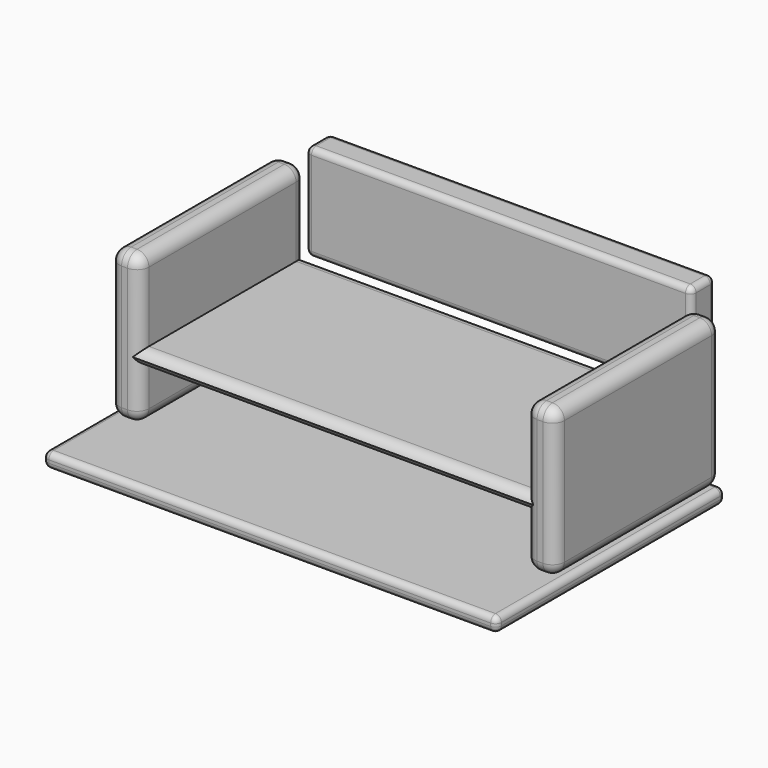
from build123d import *

# Parameters (mm, degrees)
F1_DEPTH      = 88.9
F2_DEPTH      = 6.35
F3_DEPTH      = 6.35
F4_T1_DEPTH   = 17.145
F4_T3_DEPTH   = 165.1
F4_T5_DEPTH   = 2.54
F4_T7_DEPTH   = 53.34
F4_T9_DEPTH   = 29.845
F4_T11_DEPTH  = 2.54
F4_T13_DEPTH  = 78.74
F4_S17_W      = 5.08
F4_S17_H      = 5.08
F4_T18_DEPTH  = 5.08
F4_S23_W      = 5.08
F4_S23_H      = 5.08
F4_T24_DEPTH  = 5.08
F4_S29_W      = 5.08
F4_S29_H      = 5.08
F4_T30_DEPTH  = 5.08
F4_S35_W      = 5.08
F4_S35_H      = 5.08
F4_T36_DEPTH  = 5.08
F4_S41_W      = 5.08
F4_S41_H      = 5.08
F4_T42_DEPTH  = 5.08
F4_S47_W      = 5.08
F4_S47_H      = 5.08
F4_T48_DEPTH  = 5.08
F4_S53_W      = 5.08
F4_S53_H      = 5.08
F4_T54_DEPTH  = 5.08
F4_S59_W      = 5.08
F4_S59_H      = 5.08
F4_T60_DEPTH  = 5.08
F4_S65_W      = 5.08
F4_S65_H      = 5.08
F4_T66_DEPTH  = 5.08
F4_S71_W      = 5.08
F4_S71_H      = 5.08
F4_T72_DEPTH  = 5.08
F4_S77_W      = 5.08
F4_S77_H      = 5.08
F4_T78_DEPTH  = 5.08
F4_S83_W      = 5.08
F4_S83_H      = 5.08
F4_T84_DEPTH  = 5.08
F4_S89_W      = 5.08
F4_S89_H      = 5.08
F4_T90_DEPTH  = 5.08
F4_S95_W      = 5.08
F4_S95_H      = 5.08
F4_T96_DEPTH  = 5.08
F4_S101_W     = 5.08
F4_S101_H     = 5.08
F4_T102_DEPTH = 5.08
F4_S107_W     = 5.08
F4_S107_H     = 5.08
F4_T108_DEPTH = 5.08
F4_T114_DEPTH = 29.845
F4_T119_DEPTH = 29.845
F4_T124_DEPTH = 42.545
F4_T129_DEPTH = 42.545
F4_T134_DEPTH = 29.845
F4_T139_DEPTH = 29.845
F4_T144_DEPTH = 42.545
F4_T149_DEPTH = 42.545
F4_T155_DEPTH = 29.845
F4_T160_DEPTH = 177.8
F4_T167_DEPTH = 177.8
F4_T171_DEPTH = 29.845
F4_T179_DEPTH = 42.545
F4_T184_DEPTH = 177.8
F4_T191_DEPTH = 177.8
F4_T195_DEPTH = 42.545
F4_T203_DEPTH = 29.845
F4_T208_DEPTH = 177.8
F4_T215_DEPTH = 29.845
F4_T220_DEPTH = 177.8
F4_T227_DEPTH = 177.8
F4_T231_DEPTH = 42.545
F4_T239_DEPTH = 42.545
F4_T244_DEPTH = 177.8
F5_DEPTH      = 122.15182
F6_DEPTH      = 8.30271
F7_DEPTH      = 8.03557
F8_R          = 2.54
F9_DEPTH      = 12.7
F10_R         = 2.54


# Not quite as in the source:
# - a fillet or chamfer that OpenCascade refuses, or shapes differently, is made with other operations: its cross-section is extruded or revolved along the edge and cut away or added


with BuildPart() as f1:
    # F0 (on Front) → F1 (new body)
    with BuildSketch(Plane.XZ):
        Polygon((82.55, -28.575), (88.9, -28.575), (88.9, 34.925), (82.55, 34.925), (82.55, 0), (-82.55, 0), (-82.55, 34.925), (-88.9, 34.925), (-88.9, -28.575), (-82.55, -28.575), (-82.55, -6.35), (82.55, -6.35), align=None)
    extrude(amount=F1_DEPTH)

    # F2 (add): a face of the model
    f2_faces = [f1.faces().sort_by_distance(p)[0] for p in [
        (-88.9, -44.45, 3.175),
    ]]
    extrude(f2_faces, amount=F2_DEPTH)

    # F3 (add): a face of the model
    f3_faces = [f1.faces().sort_by_distance(p)[0] for p in [
        (88.9, -44.45, 3.175),
    ]]
    extrude(f3_faces, amount=F3_DEPTH)

    # F4: fillet of radius 5.08 on 32 edges, made by hand

    # F4_s2 → F4_t1 (cut)
    with BuildSketch(Plane.XY.offset(-23.495)):
        with BuildLine():
            ThreePointArc((-82.55, -83.82), (-84.0378975516, -87.4121024484), (-87.63, -88.9))
            Line((-87.63, -88.9), (-82.55, -88.9))
            Line((-82.55, -88.9), (-82.55, -83.82))
        make_face()
        with BuildLine():
            ThreePointArc((87.63, -88.9), (84.0378975516, -87.4121024484), (82.55, -83.82))
            Line((82.55, -83.82), (82.55, -88.9))
            Line((82.55, -88.9), (87.63, -88.9))
        make_face()
        with BuildLine():
            ThreePointArc((-82.55, -5.08), (-84.0378975516, -1.4878975516), (-87.63, 0))
            Line((-87.63, 0), (-82.55, 0))
            Line((-82.55, 0), (-82.55, -5.08))
        make_face()
        with BuildLine():
            ThreePointArc((82.55, -5.08), (84.0378975516, -1.4878975516), (87.63, 0))
            Line((87.63, 0), (82.55, 0))
            Line((82.55, 0), (82.55, -5.08))
        make_face()
    extrude(amount=F4_T1_DEPTH, mode=Mode.SUBTRACT)

    # F4_s4 → F4_t3 (cut)
    with BuildSketch(Plane.YZ.offset(-82.55)):
        with BuildLine():
            ThreePointArc((-88.9, -1.27), (-87.4121024484, -4.8621024484), (-83.82, -6.35))
            Line((-83.82, -6.35), (-88.9, -6.35))
            Line((-88.9, -6.35), (-88.9, -1.27))
        make_face()
        with BuildLine():
            ThreePointArc((-88.9, -5.08), (-87.4121024484, -1.4878975516), (-83.82, 0))
            Line((-83.82, 0), (-88.9, 0))
            Line((-88.9, 0), (-88.9, -5.08))
        make_face()
        with BuildLine():
            ThreePointArc((0, -1.27), (-1.4878975516, -4.8621024484), (-5.08, -6.35))
            Line((-5.08, -6.35), (0, -6.35))
            Line((0, -6.35), (0, -1.27))
        make_face()
        with BuildLine():
            ThreePointArc((-5.08, 0), (-1.4878975516, -1.4878975516), (0, -5.08))
            Line((0, -5.08), (0, 0))
            Line((0, 0), (-5.08, 0))
        make_face()
    extrude(amount=F4_T3_DEPTH, mode=Mode.SUBTRACT)

    # F4_s6 → F4_t5 (cut)
    with BuildSketch(Plane.YZ.offset(87.63)):
        with BuildLine():
            ThreePointArc((-88.9, -23.495), (-87.4121024484, -27.0871024484), (-83.82, -28.575))
            Line((-83.82, -28.575), (-88.9, -28.575))
            Line((-88.9, -28.575), (-88.9, -23.495))
        make_face()
        with BuildLine():
            ThreePointArc((-88.9, 29.845), (-87.4121024484, 33.4371024484), (-83.82, 34.925))
            Line((-83.82, 34.925), (-88.9, 34.925))
            Line((-88.9, 34.925), (-88.9, 29.845))
        make_face()
        with BuildLine():
            ThreePointArc((-5.08, 34.925), (-1.4878975516, 33.4371024484), (0, 29.845))
            Line((0, 29.845), (0, 34.925))
            Line((0, 34.925), (-5.08, 34.925))
        make_face()
        with BuildLine():
            ThreePointArc((-5.08, -28.575), (-1.4878975516, -27.0871024484), (0, -23.495))
            Line((0, -23.495), (0, -28.575))
            Line((0, -28.575), (-5.08, -28.575))
        make_face()
    extrude(amount=F4_T5_DEPTH, mode=Mode.SUBTRACT)

    # F4_s8 → F4_t7 (cut)
    with BuildSketch(Plane.XY.offset(-23.495)):
        with BuildLine():
            ThreePointArc((90.17, -88.9), (93.7621024484, -87.4121024484), (95.25, -83.82))
            Line((95.25, -83.82), (95.25, -88.9))
            Line((95.25, -88.9), (90.17, -88.9))
        make_face()
        with BuildLine():
            ThreePointArc((-90.17, -88.9), (-93.7621024484, -87.4121024484), (-95.25, -83.82))
            Line((-95.25, -83.82), (-95.25, -88.9))
            Line((-95.25, -88.9), (-90.17, -88.9))
        make_face()
        with BuildLine():
            ThreePointArc((95.25, -5.08), (93.7621024484, -1.4878975516), (90.17, 0))
            Line((90.17, 0), (95.25, 0))
            Line((95.25, 0), (95.25, -5.08))
        make_face()
        with BuildLine():
            ThreePointArc((-95.25, -5.08), (-93.7621024484, -1.4878975516), (-90.17, 0))
            Line((-90.17, 0), (-95.25, 0))
            Line((-95.25, 0), (-95.25, -5.08))
        make_face()
    extrude(amount=F4_T7_DEPTH, mode=Mode.SUBTRACT)

    # F4_s10 → F4_t9 (cut)
    with BuildSketch(Plane.XY):
        with BuildLine():
            ThreePointArc((87.63, -88.9), (84.0378975516, -87.4121024484), (82.55, -83.82))
            Line((82.55, -83.82), (82.55, -88.9))
            Line((82.55, -88.9), (87.63, -88.9))
        make_face()
        with BuildLine():
            ThreePointArc((-87.63, -88.9), (-84.0378975516, -87.4121024484), (-82.55, -83.82))
            Line((-82.55, -83.82), (-82.55, -88.9))
            Line((-82.55, -88.9), (-87.63, -88.9))
        make_face()
        with BuildLine():
            ThreePointArc((82.55, -5.08), (84.0378975516, -1.4878975516), (87.63, 0))
            Line((87.63, 0), (82.55, 0))
            Line((82.55, 0), (82.55, -5.08))
        make_face()
        with BuildLine():
            ThreePointArc((-82.55, -5.08), (-84.0378975516, -1.4878975516), (-87.63, 0))
            Line((-87.63, 0), (-82.55, 0))
            Line((-82.55, 0), (-82.55, -5.08))
        make_face()
    extrude(amount=F4_T9_DEPTH, mode=Mode.SUBTRACT)

    # F4_s12 → F4_t11 (cut)
    with BuildSketch(Plane.YZ.offset(-90.17)):
        with BuildLine():
            ThreePointArc((-88.9, 29.845), (-87.4121024484, 33.4371024484), (-83.82, 34.925))
            Line((-83.82, 34.925), (-88.9, 34.925))
            Line((-88.9, 34.925), (-88.9, 29.845))
        make_face()
        with BuildLine():
            ThreePointArc((-88.9, -23.495), (-87.4121024484, -27.0871024484), (-83.82, -28.575))
            Line((-83.82, -28.575), (-88.9, -28.575))
            Line((-88.9, -28.575), (-88.9, -23.495))
        make_face()
        with BuildLine():
            ThreePointArc((-5.08, 34.925), (-1.4878975516, 33.4371024484), (0, 29.845))
            Line((0, 29.845), (0, 34.925))
            Line((0, 34.925), (-5.08, 34.925))
        make_face()
        with BuildLine():
            ThreePointArc((0, -23.495), (-1.4878975516, -27.0871024484), (-5.08, -28.575))
            Line((-5.08, -28.575), (0, -28.575))
            Line((0, -28.575), (0, -23.495))
        make_face()
    extrude(amount=F4_T11_DEPTH, mode=Mode.SUBTRACT)

    # F4_s14 → F4_t13 (cut)
    with BuildSketch(Plane.XZ.offset(5.08)):
        with BuildLine():
            ThreePointArc((-87.63, 34.925), (-84.0378975516, 33.4371024484), (-82.55, 29.845))
            Line((-82.55, 29.845), (-82.55, 34.925))
            Line((-82.55, 34.925), (-87.63, 34.925))
        make_face()
        with BuildLine():
            ThreePointArc((-95.25, 29.845), (-93.7621024484, 33.4371024484), (-90.17, 34.925))
            Line((-90.17, 34.925), (-95.25, 34.925))
            Line((-95.25, 34.925), (-95.25, 29.845))
        make_face()
        with BuildLine():
            ThreePointArc((82.55, 29.845), (84.0378975516, 33.4371024484), (87.63, 34.925))
            Line((87.63, 34.925), (82.55, 34.925))
            Line((82.55, 34.925), (82.55, 29.845))
        make_face()
        with BuildLine():
            ThreePointArc((90.17, 34.925), (93.7621024484, 33.4371024484), (95.25, 29.845))
            Line((95.25, 29.845), (95.25, 34.925))
            Line((95.25, 34.925), (90.17, 34.925))
        make_face()
        with BuildLine():
            ThreePointArc((87.63, -28.575), (84.0378975516, -27.0871024484), (82.55, -23.495))
            Line((82.55, -23.495), (82.55, -28.575))
            Line((82.55, -28.575), (87.63, -28.575))
        make_face()
        with BuildLine():
            ThreePointArc((95.25, -23.495), (93.7621024484, -27.0871024484), (90.17, -28.575))
            Line((90.17, -28.575), (95.25, -28.575))
            Line((95.25, -28.575), (95.25, -23.495))
        make_face()
        with BuildLine():
            ThreePointArc((-82.55, -23.495), (-84.0378975516, -27.0871024484), (-87.63, -28.575))
            Line((-87.63, -28.575), (-82.55, -28.575))
            Line((-82.55, -28.575), (-82.55, -23.495))
        make_face()
        with BuildLine():
            ThreePointArc((-95.25, -23.495), (-93.7621024484, -27.0871024484), (-90.17, -28.575))
            Line((-90.17, -28.575), (-95.25, -28.575))
            Line((-95.25, -28.575), (-95.25, -23.495))
        make_face()
    extrude(amount=F4_T13_DEPTH, mode=Mode.SUBTRACT)


with BuildPart() as f4_tool16:
    # F4_s17 → F4_t18 (new body)
    with BuildSketch(Plane.YZ.offset(-87.63)):
        with Locations((-86.36, -26.035)):
            Rectangle(F4_S17_W, F4_S17_H)
    extrude(amount=F4_T18_DEPTH)

    # F4_s19 → F4_t20 (revolve, cut)
    with BuildSketch(Plane(origin=(-87.63, -83.82, -23.495), x_dir=(0, 0.7071067812, 0.7071067812), z_dir=(0, 0.7071067812, -0.7071067812))):
        with BuildLine():
            ThreePointArc((0, -5.08), (5.08, 0), (0, 5.08))
            Line((0, 5.08), (0, -5.08))
        make_face()
    revolve(axis=Axis((-87.63, -83.82, -23.495), (1, 0, 0)), mode=Mode.SUBTRACT)


with BuildPart() as f1_1:
    add(f1.part)

    # F4_t15: cut F4_tool16
    add(f4_tool16.part, mode=Mode.SUBTRACT)


with BuildPart() as f4_tool22:
    # F4_s23 → F4_t24 (new body)
    with BuildSketch(Plane.XZ.offset(83.82)):
        with Locations((85.09, -26.035)):
            Rectangle(F4_S23_W, F4_S23_H)
    extrude(amount=F4_T24_DEPTH)

    # F4_s25 → F4_t26 (revolve, cut)
    with BuildSketch(Plane(origin=(87.63, -83.82, -23.495), x_dir=(0.7071067812, 0, 0.7071067812), z_dir=(0.7071067812, 0, -0.7071067812))):
        with BuildLine():
            ThreePointArc((0, -5.08), (5.08, 0), (0, 5.08))
            Line((0, 5.08), (0, -5.08))
        make_face()
    revolve(axis=Axis((87.63, -83.82, -23.495), (0, -1, 0)), mode=Mode.SUBTRACT)


with BuildPart() as f1_2:
    add(f1_1.part)

    # F4_t21: cut F4_tool22
    add(f4_tool22.part, mode=Mode.SUBTRACT)


with BuildPart() as f4_tool28:
    # F4_s29 → F4_t30 (new body)
    with BuildSketch(Plane.YZ.offset(90.17)):
        with Locations((-86.36, -26.035)):
            Rectangle(F4_S29_W, F4_S29_H)
    extrude(amount=F4_T30_DEPTH)

    # F4_s31 → F4_t32 (revolve, cut)
    with BuildSketch(Plane(origin=(90.17, -83.82, -23.495), x_dir=(0, 0.7071067812, 0.7071067812), z_dir=(0, 0.7071067812, -0.7071067812))):
        with BuildLine():
            ThreePointArc((0, -5.08), (5.08, 0), (0, 5.08))
            Line((0, 5.08), (0, -5.08))
        make_face()
    revolve(axis=Axis((90.17, -83.82, -23.495), (1, 0, 0)), mode=Mode.SUBTRACT)


with BuildPart() as f1_3:
    add(f1_2.part)

    # F4_t27: cut F4_tool28
    add(f4_tool28.part, mode=Mode.SUBTRACT)


with BuildPart() as f4_tool34:
    # F4_s35 → F4_t36 (new body)
    with BuildSketch(Plane.YZ.offset(90.17)):
        with Locations((-86.36, 32.385)):
            Rectangle(F4_S35_W, F4_S35_H)
    extrude(amount=F4_T36_DEPTH)

    # F4_s37 → F4_t38 (revolve, cut)
    with BuildSketch(Plane(origin=(90.17, -83.82, 29.845), x_dir=(0, 0.7071067812, -0.7071067812), z_dir=(0, -0.7071067812, -0.7071067812))):
        with BuildLine():
            ThreePointArc((0, -5.08), (5.08, 0), (0, 5.08))
            Line((0, 5.08), (0, -5.08))
        make_face()
    revolve(axis=Axis((90.17, -83.82, 29.845), (1, 0, 0)), mode=Mode.SUBTRACT)


with BuildPart() as f1_4:
    add(f1_3.part)

    # F4_t33: cut F4_tool34
    add(f4_tool34.part, mode=Mode.SUBTRACT)


with BuildPart() as f4_tool40:
    # F4_s41 → F4_t42 (new body)
    with BuildSketch(Plane.XZ.offset(83.82)):
        with Locations((85.09, 32.385)):
            Rectangle(F4_S41_W, F4_S41_H)
    extrude(amount=F4_T42_DEPTH)

    # F4_s43 → F4_t44 (revolve, cut)
    with BuildSketch(Plane(origin=(87.63, -83.82, 29.845), x_dir=(0.7071067812, 0, -0.7071067812), z_dir=(-0.7071067812, 0, -0.7071067812))):
        with BuildLine():
            ThreePointArc((0, -5.08), (5.08, 0), (0, 5.08))
            Line((0, 5.08), (0, -5.08))
        make_face()
    revolve(axis=Axis((87.63, -83.82, 29.845), (0, -1, 0)), mode=Mode.SUBTRACT)


with BuildPart() as f1_5:
    add(f1_4.part)

    # F4_t39: cut F4_tool40
    add(f4_tool40.part, mode=Mode.SUBTRACT)


with BuildPart() as f4_tool46:
    # F4_s47 → F4_t48 (new body)
    with BuildSketch(Plane.XZ.offset(83.82)):
        with Locations((-85.09, 32.385)):
            Rectangle(F4_S47_W, F4_S47_H)
    extrude(amount=F4_T48_DEPTH)

    # F4_s49 → F4_t50 (revolve, cut)
    with BuildSketch(Plane(origin=(-87.63, -83.82, 29.845), x_dir=(-0.7071067812, 0, -0.7071067812), z_dir=(-0.7071067812, 0, 0.7071067812))):
        with BuildLine():
            ThreePointArc((0, -5.08), (5.08, 0), (0, 5.08))
            Line((0, 5.08), (0, -5.08))
        make_face()
    revolve(axis=Axis((-87.63, -83.82, 29.845), (0, -1, 0)), mode=Mode.SUBTRACT)


with BuildPart() as f1_6:
    add(f1_5.part)

    # F4_t45: cut F4_tool46
    add(f4_tool46.part, mode=Mode.SUBTRACT)


with BuildPart() as f4_tool52:
    # F4_s53 → F4_t54 (new body)
    with BuildSketch(Plane.XZ.offset(83.82)):
        with Locations((-92.71, 32.385)):
            Rectangle(F4_S53_W, F4_S53_H)
    extrude(amount=F4_T54_DEPTH)

    # F4_s55 → F4_t56 (revolve, cut)
    with BuildSketch(Plane(origin=(-90.17, -83.82, 29.845), x_dir=(0.7071067812, 0, -0.7071067812), z_dir=(-0.7071067812, 0, -0.7071067812))):
        with BuildLine():
            ThreePointArc((0, -5.08), (5.08, 0), (0, 5.08))
            Line((0, 5.08), (0, -5.08))
        make_face()
    revolve(axis=Axis((-90.17, -83.82, 29.845), (0, -1, 0)), mode=Mode.SUBTRACT)


with BuildPart() as f1_7:
    add(f1_6.part)

    # F4_t51: cut F4_tool52
    add(f4_tool52.part, mode=Mode.SUBTRACT)


with BuildPart() as f4_tool58:
    # F4_s59 → F4_t60 (new body)
    with BuildSketch(Plane.XZ.offset(83.82)):
        with Locations((-92.71, -26.035)):
            Rectangle(F4_S59_W, F4_S59_H)
    extrude(amount=F4_T60_DEPTH)

    # F4_s61 → F4_t62 (revolve, cut)
    with BuildSketch(Plane(origin=(-90.17, -83.82, -23.495), x_dir=(0.7071067812, 0, 0.7071067812), z_dir=(0.7071067812, 0, -0.7071067812))):
        with BuildLine():
            ThreePointArc((0, -5.08), (5.08, 0), (0, 5.08))
            Line((0, 5.08), (0, -5.08))
        make_face()
    revolve(axis=Axis((-90.17, -83.82, -23.495), (0, -1, 0)), mode=Mode.SUBTRACT)


with BuildPart() as f1_8:
    add(f1_7.part)

    # F4_t57: cut F4_tool58
    add(f4_tool58.part, mode=Mode.SUBTRACT)


with BuildPart() as f4_tool64:
    # F4_s65 → F4_t66 (new body)
    with BuildSketch(Plane.XZ.offset(5.08)):
        with Locations((-85.09, 32.385)):
            Rectangle(F4_S65_W, F4_S65_H)
    extrude(amount=-F4_T66_DEPTH)

    # F4_s67 → F4_t68 (revolve, cut)
    with BuildSketch(Plane(origin=(-87.63, -5.08, 29.845), x_dir=(-0.7071067812, 0, -0.7071067812), z_dir=(0.7071067812, 0, -0.7071067812))):
        with BuildLine():
            ThreePointArc((0, -5.08), (5.08, 0), (0, 5.08))
            Line((0, 5.08), (0, -5.08))
        make_face()
    revolve(axis=Axis((-87.63, -5.08, 29.845), (0, 1, 0)), mode=Mode.SUBTRACT)


with BuildPart() as f1_9:
    add(f1_8.part)

    # F4_t63: cut F4_tool64
    add(f4_tool64.part, mode=Mode.SUBTRACT)


with BuildPart() as f4_tool70:
    # F4_s71 → F4_t72 (new body)
    with BuildSketch(Plane.XZ.offset(5.08)):
        with Locations((-92.71, 32.385)):
            Rectangle(F4_S71_W, F4_S71_H)
    extrude(amount=-F4_T72_DEPTH)

    # F4_s73 → F4_t74 (revolve, cut)
    with BuildSketch(Plane(origin=(-90.17, -5.08, 29.845), x_dir=(0.7071067812, 0, -0.7071067812), z_dir=(0.7071067812, 0, 0.7071067812))):
        with BuildLine():
            ThreePointArc((0, -5.08), (5.08, 0), (0, 5.08))
            Line((0, 5.08), (0, -5.08))
        make_face()
    revolve(axis=Axis((-90.17, -5.08, 29.845), (0, 1, 0)), mode=Mode.SUBTRACT)


with BuildPart() as f1_10:
    add(f1_9.part)

    # F4_t69: cut F4_tool70
    add(f4_tool70.part, mode=Mode.SUBTRACT)


with BuildPart() as f4_tool76:
    # F4_s77 → F4_t78 (new body)
    with BuildSketch(Plane.XZ.offset(5.08)):
        with Locations((85.09, 32.385)):
            Rectangle(F4_S77_W, F4_S77_H)
    extrude(amount=-F4_T78_DEPTH)

    # F4_s79 → F4_t80 (revolve, cut)
    with BuildSketch(Plane(origin=(87.63, -5.08, 29.845), x_dir=(0.7071067812, 0, -0.7071067812), z_dir=(0.7071067812, 0, 0.7071067812))):
        with BuildLine():
            ThreePointArc((0, -5.08), (5.08, 0), (0, 5.08))
            Line((0, 5.08), (0, -5.08))
        make_face()
    revolve(axis=Axis((87.63, -5.08, 29.845), (0, 1, 0)), mode=Mode.SUBTRACT)


with BuildPart() as f1_11:
    add(f1_10.part)

    # F4_t75: cut F4_tool76
    add(f4_tool76.part, mode=Mode.SUBTRACT)


with BuildPart() as f4_tool82:
    # F4_s83 → F4_t84 (new body)
    with BuildSketch(Plane.YZ.offset(90.17)):
        with Locations((-2.54, 32.385)):
            Rectangle(F4_S83_W, F4_S83_H)
    extrude(amount=F4_T84_DEPTH)

    # F4_s85 → F4_t86 (revolve, cut)
    with BuildSketch(Plane(origin=(90.17, -5.08, 29.845), x_dir=(0, -0.7071067812, -0.7071067812), z_dir=(0, -0.7071067812, 0.7071067812))):
        with BuildLine():
            ThreePointArc((0, -5.08), (5.08, 0), (0, 5.08))
            Line((0, 5.08), (0, -5.08))
        make_face()
    revolve(axis=Axis((90.17, -5.08, 29.845), (1, 0, 0)), mode=Mode.SUBTRACT)


with BuildPart() as f1_12:
    add(f1_11.part)

    # F4_t81: cut F4_tool82
    add(f4_tool82.part, mode=Mode.SUBTRACT)


with BuildPart() as f4_tool88:
    # F4_s89 → F4_t90 (new body)
    with BuildSketch(Plane.XY.offset(-23.495)):
        with Locations((85.09, -2.54)):
            Rectangle(F4_S89_W, F4_S89_H)
    extrude(amount=-F4_T90_DEPTH)

    # F4_s91 → F4_t92 (revolve, cut)
    with BuildSketch(Plane(origin=(87.63, -5.08, -23.495), x_dir=(0.7071067812, -0.7071067812, 0), z_dir=(0.7071067812, 0.7071067812, 0))):
        with BuildLine():
            ThreePointArc((0, -5.08), (5.08, 0), (0, 5.08))
            Line((0, 5.08), (0, -5.08))
        make_face()
    revolve(axis=Axis((87.63, -5.08, -23.495), (0, 0, -1)), mode=Mode.SUBTRACT)


with BuildPart() as f1_13:
    add(f1_12.part)

    # F4_t87: cut F4_tool88
    add(f4_tool88.part, mode=Mode.SUBTRACT)


with BuildPart() as f4_tool94:
    # F4_s95 → F4_t96 (new body)
    with BuildSketch(Plane.YZ.offset(90.17)):
        with Locations((-2.54, -26.035)):
            Rectangle(F4_S95_W, F4_S95_H)
    extrude(amount=F4_T96_DEPTH)

    # F4_s97 → F4_t98 (revolve, cut)
    with BuildSketch(Plane(origin=(90.17, -5.08, -23.495), x_dir=(0, -0.7071067812, 0.7071067812), z_dir=(0, 0.7071067812, 0.7071067812))):
        with BuildLine():
            ThreePointArc((0, -5.08), (5.08, 0), (0, 5.08))
            Line((0, 5.08), (0, -5.08))
        make_face()
    revolve(axis=Axis((90.17, -5.08, -23.495), (1, 0, 0)), mode=Mode.SUBTRACT)


with BuildPart() as f1_14:
    add(f1_13.part)

    # F4_t93: cut F4_tool94
    add(f4_tool94.part, mode=Mode.SUBTRACT)


with BuildPart() as f4_tool100:
    # F4_s101 → F4_t102 (new body)
    with BuildSketch(Plane.YZ.offset(-87.63)):
        with Locations((-2.54, -26.035)):
            Rectangle(F4_S101_W, F4_S101_H)
    extrude(amount=F4_T102_DEPTH)

    # F4_s103 → F4_t104 (revolve, cut)
    with BuildSketch(Plane(origin=(-87.63, -5.08, -23.495), x_dir=(0, -0.7071067812, 0.7071067812), z_dir=(0, 0.7071067812, 0.7071067812))):
        with BuildLine():
            ThreePointArc((0, -5.08), (5.08, 0), (0, 5.08))
            Line((0, 5.08), (0, -5.08))
        make_face()
    revolve(axis=Axis((-87.63, -5.08, -23.495), (1, 0, 0)), mode=Mode.SUBTRACT)


with BuildPart() as f1_15:
    add(f1_14.part)

    # F4_t99: cut F4_tool100
    add(f4_tool100.part, mode=Mode.SUBTRACT)


with BuildPart() as f4_tool106:
    # F4_s107 → F4_t108 (new body)
    with BuildSketch(Plane.YZ.offset(-90.17)):
        with Locations((-2.54, -26.035)):
            Rectangle(F4_S107_W, F4_S107_H)
    extrude(amount=-F4_T108_DEPTH)

    # F4_s109 → F4_t110 (revolve, cut)
    with BuildSketch(Plane(origin=(-90.17, -5.08, -23.495), x_dir=(0, -0.7071067812, 0.7071067812), z_dir=(0, -0.7071067812, -0.7071067812))):
        with BuildLine():
            ThreePointArc((0, -5.08), (5.08, 0), (0, 5.08))
            Line((0, 5.08), (0, -5.08))
        make_face()
    revolve(axis=Axis((-90.17, -5.08, -23.495), (-1, 0, 0)), mode=Mode.SUBTRACT)


with BuildPart() as f1_16:
    add(f1_15.part)

    # F4_t105: cut F4_tool106
    add(f4_tool106.part, mode=Mode.SUBTRACT)


with BuildPart() as f4_tool112:
    # F4_s113 → F4_t114 (new body)
    with BuildSketch(Plane.XY.offset(-23.495)):
        with BuildLine():
            ThreePointArc((-82.55, -83.82), (-84.0378975516, -87.4121024484), (-87.63, -88.9))
            Line((-87.63, -88.9), (-82.55, -88.9))
            Line((-82.55, -88.9), (-82.55, -83.82))
        make_face()
    extrude(amount=F4_T114_DEPTH)

    split(bisect_by=Plane.XY, keep=Keep.TOP)


with BuildPart() as f1_17:
    add(f1_16.part)

    # F4_t111: cut F4_tool112
    add(f4_tool112.part, mode=Mode.SUBTRACT)


with BuildPart() as f4_tool117:
    # F4_s118 → F4_t119 (new body)
    with BuildSketch(Plane.XY.offset(6.35)):
        with BuildLine():
            ThreePointArc((87.63, -88.9), (84.0378975516, -87.4121024484), (82.55, -83.82))
            Line((82.55, -83.82), (82.55, -88.9))
            Line((82.55, -88.9), (87.63, -88.9))
        make_face()
    extrude(amount=-F4_T119_DEPTH)

    split(bisect_by=Plane.XY, keep=Keep.TOP)


with BuildPart() as f1_18:
    add(f1_17.part)

    # F4_t116: cut F4_tool117
    add(f4_tool117.part, mode=Mode.SUBTRACT)


with BuildPart() as f4_tool122:
    # F4_s123 → F4_t124 (new body)
    with BuildSketch(Plane.XY.offset(29.845)):
        with BuildLine():
            ThreePointArc((87.63, -88.9), (84.0378975516, -87.4121024484), (82.55, -83.82))
            Line((82.55, -83.82), (82.55, -88.9))
            Line((82.55, -88.9), (87.63, -88.9))
        make_face()
    extrude(amount=-F4_T124_DEPTH)

    split(bisect_by=Plane.XY.offset(-6.35), keep=Keep.BOTTOM)


with BuildPart() as f1_19:
    add(f1_18.part)

    # F4_t121: cut F4_tool122
    add(f4_tool122.part, mode=Mode.SUBTRACT)


with BuildPart() as f4_tool127:
    # F4_s128 → F4_t129 (new body)
    with BuildSketch(Plane.XY.offset(-12.7)):
        with BuildLine():
            ThreePointArc((-87.63, -88.9), (-84.0378975516, -87.4121024484), (-82.55, -83.82))
            Line((-82.55, -83.82), (-82.55, -88.9))
            Line((-82.55, -88.9), (-87.63, -88.9))
        make_face()
    extrude(amount=F4_T129_DEPTH)

    split(bisect_by=Plane.XY.offset(-6.35), keep=Keep.BOTTOM)


with BuildPart() as f1_20:
    add(f1_19.part)

    # F4_t126: cut F4_tool127
    add(f4_tool127.part, mode=Mode.SUBTRACT)


with BuildPart() as f4_tool132:
    # F4_s133 → F4_t134 (new body)
    with BuildSketch(Plane.XY.offset(-23.495)):
        with BuildLine():
            ThreePointArc((-82.55, -5.08), (-84.0378975516, -1.4878975516), (-87.63, 0))
            Line((-87.63, 0), (-82.55, 0))
            Line((-82.55, 0), (-82.55, -5.08))
        make_face()
    extrude(amount=F4_T134_DEPTH)

    split(bisect_by=Plane.XY, keep=Keep.TOP)


with BuildPart() as f1_21:
    add(f1_20.part)

    # F4_t131: cut F4_tool132
    add(f4_tool132.part, mode=Mode.SUBTRACT)


with BuildPart() as f4_tool137:
    # F4_s138 → F4_t139 (new body)
    with BuildSketch(Plane.XY.offset(6.35)):
        with BuildLine():
            ThreePointArc((82.55, -5.08), (84.0378975516, -1.4878975516), (87.63, 0))
            Line((87.63, 0), (82.55, 0))
            Line((82.55, 0), (82.55, -5.08))
        make_face()
    extrude(amount=-F4_T139_DEPTH)

    split(bisect_by=Plane.XY, keep=Keep.TOP)


with BuildPart() as f1_22:
    add(f1_21.part)

    # F4_t136: cut F4_tool137
    add(f4_tool137.part, mode=Mode.SUBTRACT)


with BuildPart() as f4_tool142:
    # F4_s143 → F4_t144 (new body)
    with BuildSketch(Plane.XY.offset(29.845)):
        with BuildLine():
            ThreePointArc((82.55, -5.08), (84.0378975516, -1.4878975516), (87.63, 0))
            Line((87.63, 0), (82.55, 0))
            Line((82.55, 0), (82.55, -5.08))
        make_face()
    extrude(amount=-F4_T144_DEPTH)

    split(bisect_by=Plane.XY.offset(-6.35), keep=Keep.BOTTOM)


with BuildPart() as f1_23:
    add(f1_22.part)

    # F4_t141: cut F4_tool142
    add(f4_tool142.part, mode=Mode.SUBTRACT)


with BuildPart() as f4_tool147:
    # F4_s148 → F4_t149 (new body)
    with BuildSketch(Plane.XY.offset(-12.7)):
        with BuildLine():
            ThreePointArc((-82.55, -5.08), (-84.0378975516, -1.4878975516), (-87.63, 0))
            Line((-87.63, 0), (-82.55, 0))
            Line((-82.55, 0), (-82.55, -5.08))
        make_face()
    extrude(amount=F4_T149_DEPTH)

    split(bisect_by=Plane.XY.offset(-6.35), keep=Keep.BOTTOM)


with BuildPart() as f1_24:
    add(f1_23.part)

    # F4_t146: cut F4_tool147
    add(f4_tool147.part, mode=Mode.SUBTRACT)


with BuildPart() as f4_tool153:
    # F4_s154 → F4_t155 (new body)
    with BuildSketch(Plane.XY.offset(-23.495)):
        with BuildLine():
            ThreePointArc((-82.55, -83.82), (-84.0378975516, -87.4121024484), (-87.63, -88.9))
            Line((-87.63, -88.9), (-82.55, -88.9))
            Line((-82.55, -88.9), (-82.55, -83.82))
        make_face()
    extrude(amount=F4_T155_DEPTH)

    split(bisect_by=Plane.XY.offset(-6.35), keep=Keep.TOP)

    split(bisect_by=Plane.XY, keep=Keep.BOTTOM)


with BuildPart() as f4_tool158:
    # F4_s159 → F4_t160 (new body)
    with BuildSketch(Plane.YZ.offset(-95.25)):
        with BuildLine():
            ThreePointArc((-88.9, -1.27), (-87.4121024484, -4.8621024484), (-83.82, -6.35))
            Line((-83.82, -6.35), (-88.9, -6.35))
            Line((-88.9, -6.35), (-88.9, -1.27))
        make_face()
    extrude(amount=F4_T160_DEPTH)

    split(bisect_by=Plane.YZ.offset(-82.55), keep=Keep.BOTTOM)


with BuildPart() as f4_tool153_1:
    add(f4_tool153.part)

    # F4_t162: intersect F4_tool158
    add(f4_tool158.part, mode=Mode.INTERSECT)


with BuildPart() as f1_25:
    add(f1_24.part)

    # F4_t151: cut F4_tool153
    add(f4_tool153_1.part, mode=Mode.SUBTRACT)


with BuildPart() as f4_tool165:
    # F4_s166 → F4_t167 (new body)
    with BuildSketch(Plane.YZ.offset(-82.55)):
        with BuildLine():
            ThreePointArc((-88.9, -1.27), (-87.4121024484, -4.8621024484), (-83.82, -6.35))
            Line((-83.82, -6.35), (-88.9, -6.35))
            Line((-88.9, -6.35), (-88.9, -1.27))
        make_face()
    extrude(amount=F4_T167_DEPTH)

    split(bisect_by=Plane.YZ.offset(82.55), keep=Keep.TOP)


with BuildPart() as f4_tool169:
    # F4_s170 → F4_t171 (new body)
    with BuildSketch(Plane.XY.offset(6.35)):
        with BuildLine():
            ThreePointArc((87.63, -88.9), (84.0378975516, -87.4121024484), (82.55, -83.82))
            Line((82.55, -83.82), (82.55, -88.9))
            Line((82.55, -88.9), (87.63, -88.9))
        make_face()
    extrude(amount=-F4_T171_DEPTH)

    split(bisect_by=Plane.XY, keep=Keep.BOTTOM)

    split(bisect_by=Plane.XY.offset(-6.35), keep=Keep.TOP)


with BuildPart() as f4_tool165_1:
    add(f4_tool165.part)

    # F4_t174: intersect F4_tool169
    add(f4_tool169.part, mode=Mode.INTERSECT)


with BuildPart() as f1_26:
    add(f1_25.part)

    # F4_t163: cut F4_tool165
    add(f4_tool165_1.part, mode=Mode.SUBTRACT)


with BuildPart() as f4_tool177:
    # F4_s178 → F4_t179 (new body)
    with BuildSketch(Plane.XY.offset(29.845)):
        with BuildLine():
            ThreePointArc((87.63, -88.9), (84.0378975516, -87.4121024484), (82.55, -83.82))
            Line((82.55, -83.82), (82.55, -88.9))
            Line((82.55, -88.9), (87.63, -88.9))
        make_face()
    extrude(amount=-F4_T179_DEPTH)

    split(bisect_by=Plane.XY, keep=Keep.BOTTOM)

    split(bisect_by=Plane.XY.offset(-6.35), keep=Keep.TOP)


with BuildPart() as f4_tool182:
    # F4_s183 → F4_t184 (new body)
    with BuildSketch(Plane.YZ.offset(95.25)):
        with BuildLine():
            ThreePointArc((-88.9, -5.08), (-87.4121024484, -1.4878975516), (-83.82, 0))
            Line((-83.82, 0), (-88.9, 0))
            Line((-88.9, 0), (-88.9, -5.08))
        make_face()
    extrude(amount=-F4_T184_DEPTH)

    split(bisect_by=Plane.YZ.offset(82.55), keep=Keep.TOP)


with BuildPart() as f4_tool177_1:
    add(f4_tool177.part)

    # F4_t186: intersect F4_tool182
    add(f4_tool182.part, mode=Mode.INTERSECT)


with BuildPart() as f1_27:
    add(f1_26.part)

    # F4_t175: cut F4_tool177
    add(f4_tool177_1.part, mode=Mode.SUBTRACT)


with BuildPart() as f4_tool189:
    # F4_s190 → F4_t191 (new body)
    with BuildSketch(Plane.YZ.offset(82.55)):
        with BuildLine():
            ThreePointArc((-88.9, -5.08), (-87.4121024484, -1.4878975516), (-83.82, 0))
            Line((-83.82, 0), (-88.9, 0))
            Line((-88.9, 0), (-88.9, -5.08))
        make_face()
    extrude(amount=-F4_T191_DEPTH)

    split(bisect_by=Plane.YZ.offset(-82.55), keep=Keep.BOTTOM)


with BuildPart() as f4_tool193:
    # F4_s194 → F4_t195 (new body)
    with BuildSketch(Plane.XY.offset(-12.7)):
        with BuildLine():
            ThreePointArc((-87.63, -88.9), (-84.0378975516, -87.4121024484), (-82.55, -83.82))
            Line((-82.55, -83.82), (-82.55, -88.9))
            Line((-82.55, -88.9), (-87.63, -88.9))
        make_face()
    extrude(amount=F4_T195_DEPTH)

    split(bisect_by=Plane.XY.offset(-6.35), keep=Keep.TOP)

    split(bisect_by=Plane.XY, keep=Keep.BOTTOM)


with BuildPart() as f4_tool189_1:
    add(f4_tool189.part)

    # F4_t198: intersect F4_tool193
    add(f4_tool193.part, mode=Mode.INTERSECT)


with BuildPart() as f1_28:
    add(f1_27.part)

    # F4_t187: cut F4_tool189
    add(f4_tool189_1.part, mode=Mode.SUBTRACT)


with BuildPart() as f4_tool201:
    # F4_s202 → F4_t203 (new body)
    with BuildSketch(Plane.XY.offset(-23.495)):
        with BuildLine():
            ThreePointArc((-82.55, -5.08), (-84.0378975516, -1.4878975516), (-87.63, 0))
            Line((-87.63, 0), (-82.55, 0))
            Line((-82.55, 0), (-82.55, -5.08))
        make_face()
    extrude(amount=F4_T203_DEPTH)

    split(bisect_by=Plane.XY.offset(-6.35), keep=Keep.TOP)

    split(bisect_by=Plane.XY, keep=Keep.BOTTOM)


with BuildPart() as f4_tool206:
    # F4_s207 → F4_t208 (new body)
    with BuildSketch(Plane.YZ.offset(-95.25)):
        with BuildLine():
            ThreePointArc((0, -1.27), (-1.4878975516, -4.8621024484), (-5.08, -6.35))
            Line((-5.08, -6.35), (0, -6.35))
            Line((0, -6.35), (0, -1.27))
        make_face()
    extrude(amount=F4_T208_DEPTH)

    split(bisect_by=Plane.YZ.offset(-82.55), keep=Keep.BOTTOM)


with BuildPart() as f4_tool201_1:
    add(f4_tool201.part)

    # F4_t210: intersect F4_tool206
    add(f4_tool206.part, mode=Mode.INTERSECT)


with BuildPart() as f1_29:
    add(f1_28.part)

    # F4_t199: cut F4_tool201
    add(f4_tool201_1.part, mode=Mode.SUBTRACT)


with BuildPart() as f4_tool213:
    # F4_s214 → F4_t215 (new body)
    with BuildSketch(Plane.XY.offset(6.35)):
        with BuildLine():
            ThreePointArc((82.55, -5.08), (84.0378975516, -1.4878975516), (87.63, 0))
            Line((87.63, 0), (82.55, 0))
            Line((82.55, 0), (82.55, -5.08))
        make_face()
    extrude(amount=-F4_T215_DEPTH)

    split(bisect_by=Plane.XY, keep=Keep.BOTTOM)

    split(bisect_by=Plane.XY.offset(-6.35), keep=Keep.TOP)


with BuildPart() as f4_tool218:
    # F4_s219 → F4_t220 (new body)
    with BuildSketch(Plane.YZ.offset(-82.55)):
        with BuildLine():
            ThreePointArc((0, -1.27), (-1.4878975516, -4.8621024484), (-5.08, -6.35))
            Line((-5.08, -6.35), (0, -6.35))
            Line((0, -6.35), (0, -1.27))
        make_face()
    extrude(amount=F4_T220_DEPTH)

    split(bisect_by=Plane.YZ.offset(82.55), keep=Keep.TOP)


with BuildPart() as f4_tool213_1:
    add(f4_tool213.part)

    # F4_t222: intersect F4_tool218
    add(f4_tool218.part, mode=Mode.INTERSECT)


with BuildPart() as f1_30:
    add(f1_29.part)

    # F4_t211: cut F4_tool213
    add(f4_tool213_1.part, mode=Mode.SUBTRACT)


with BuildPart() as f4_tool225:
    # F4_s226 → F4_t227 (new body)
    with BuildSketch(Plane.YZ.offset(95.25)):
        with BuildLine():
            ThreePointArc((-5.08, 0), (-1.4878975516, -1.4878975516), (0, -5.08))
            Line((0, -5.08), (0, 0))
            Line((0, 0), (-5.08, 0))
        make_face()
    extrude(amount=-F4_T227_DEPTH)

    split(bisect_by=Plane.YZ.offset(82.55), keep=Keep.TOP)


with BuildPart() as f4_tool229:
    # F4_s230 → F4_t231 (new body)
    with BuildSketch(Plane.XY.offset(29.845)):
        with BuildLine():
            ThreePointArc((82.55, -5.08), (84.0378975516, -1.4878975516), (87.63, 0))
            Line((87.63, 0), (82.55, 0))
            Line((82.55, 0), (82.55, -5.08))
        make_face()
    extrude(amount=-F4_T231_DEPTH)

    split(bisect_by=Plane.XY, keep=Keep.BOTTOM)

    split(bisect_by=Plane.XY.offset(-6.35), keep=Keep.TOP)


with BuildPart() as f4_tool225_1:
    add(f4_tool225.part)

    # F4_t234: intersect F4_tool229
    add(f4_tool229.part, mode=Mode.INTERSECT)


with BuildPart() as f1_31:
    add(f1_30.part)

    # F4_t223: cut F4_tool225
    add(f4_tool225_1.part, mode=Mode.SUBTRACT)


with BuildPart() as f4_tool237:
    # F4_s238 → F4_t239 (new body)
    with BuildSketch(Plane.XY.offset(-12.7)):
        with BuildLine():
            ThreePointArc((-82.55, -5.08), (-84.0378975516, -1.4878975516), (-87.63, 0))
            Line((-87.63, 0), (-82.55, 0))
            Line((-82.55, 0), (-82.55, -5.08))
        make_face()
    extrude(amount=F4_T239_DEPTH)

    split(bisect_by=Plane.XY.offset(-6.35), keep=Keep.TOP)

    split(bisect_by=Plane.XY, keep=Keep.BOTTOM)


with BuildPart() as f4_tool242:
    # F4_s243 → F4_t244 (new body)
    with BuildSketch(Plane.YZ.offset(82.55)):
        with BuildLine():
            ThreePointArc((-5.08, 0), (-1.4878975516, -1.4878975516), (0, -5.08))
            Line((0, -5.08), (0, 0))
            Line((0, 0), (-5.08, 0))
        make_face()
    extrude(amount=-F4_T244_DEPTH)

    split(bisect_by=Plane.YZ.offset(-82.55), keep=Keep.BOTTOM)


with BuildPart() as f4_tool237_1:
    add(f4_tool237.part)

    # F4_t246: intersect F4_tool242
    add(f4_tool242.part, mode=Mode.INTERSECT)


with BuildPart() as f1_32:
    add(f1_31.part)

    # F4_t235: cut F4_tool237
    add(f4_tool237_1.part, mode=Mode.SUBTRACT)

    # F0 (on Front) → F5 (join)
    with BuildSketch(Plane.XZ):
        Polygon((-88.9, -34.925), (88.9, -34.925), (88.9, -28.575), (82.55, -28.575), (-82.55, -28.575), (-88.9, -28.575), align=None)
    extrude(amount=F5_DEPTH)

    # F6 (add): a face of the model
    f6_faces = [f1_32.faces().sort_by_distance(p)[0] for p in [
        (-88.9, -61.07591, -31.75),
    ]]
    extrude(f6_faces, amount=F6_DEPTH)

    # F7 (add): a face of the model
    f7_faces = [f1_32.faces().sort_by_distance(p)[0] for p in [
        (88.9, -61.07591, -31.75),
    ]]
    extrude(f7_faces, amount=F7_DEPTH)

    # F8
    f8_edges = [f1_32.edges().sort_by_distance(p)[0] for p in [
        (-0.13357, -122.15182, -28.575),
        (-97.20271, -122.15182, -31.75),
        (-0.13357, -122.15182, -34.925),
        (96.93557, -122.15182, -31.75),
        (96.93557, -61.07591, -34.925),
        (96.93557, -61.07591, -28.575),
        (96.93557, 0, -31.75),
        (-97.20271, -61.07591, -28.575),
        (-97.20271, -61.07591, -34.925),
        (-97.20271, 0, -31.75),
        (-0.13357, 0, -34.925),
        (-0.13357, 0, -28.575),
    ]]
    fillet(f8_edges, radius=F8_R)


with BuildPart() as f9:
    # F0 (on Front) → F9 (new body)
    with BuildSketch(Plane.XZ):
        Polygon((82.55, 0), (82.55, 34.925), (82.55, 41.2724204361), (-82.55, 41.2724204361), (-82.55, 34.925), (-82.55, 0), align=None)
    extrude(amount=-F9_DEPTH)

    # F10
    f10_edges = [f9.edges().sort_by_distance(p)[0] for p in [
        (82.55, 6.35, 0),
        (82.55, 12.7, 20.63621),
        (82.55, 6.35, 41.27242),
        (82.55, 0, 20.63621),
        (0, 12.7, 41.27242),
        (0, 0, 41.27242),
        (-82.55, 6.35, 41.27242),
        (-82.55, 12.7, 20.63621),
        (-82.55, 0, 20.63621),
        (0, 12.7, 0),
        (0, 0, 0),
        (-82.55, 6.35, 0),
    ]]
    fillet(f10_edges, radius=F10_R)


solid = Compound([f1_32.part, f9.part])
